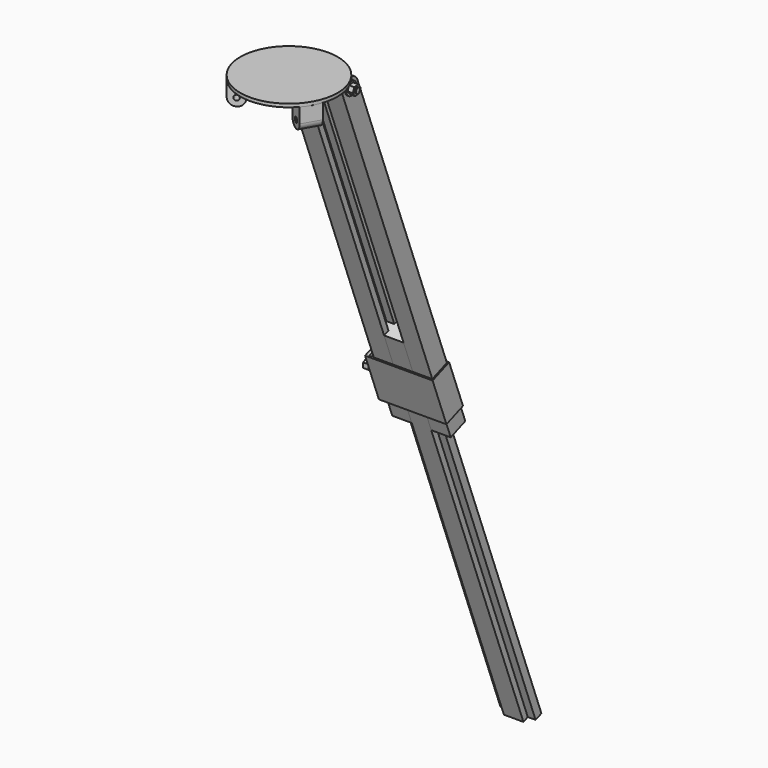
from build123d import *

# Parameters (mm, degrees)
F0_R           = 75
F1_DEPTH       = 5
F2_W           = 30
F2_H           = 24
F3_DEPTH       = 35
F4_R           = 4
F5_DEPTH       = 90.001
F6_R           = 11.99999
F7_COUNT       = 3
F8_R           = 4
F9_DEPTH       = 30
F10_R          = 14.99999
F11_W          = 24
F11_H          = 12
F12_DEPTH      = 570
F15_DEPTH      = 500
F15_DEPTH_BACK = 150
F16_R          = 10
F16_R_2        = 4
F17_DEPTH      = 2
F19_R          = 4
F20_DEPTH      = 104
F22_DEPTH      = 8
F23_R          = 4
F24_DEPTH      = 8
F26_W          = 104
F26_H          = 34
F26_W_2        = 100
F26_H_2        = 30
F27_DEPTH      = 75
F28_W          = 3
F28_H          = 30
F29_DEPTH      = 75
F30_R          = 4
F31_DEPTH      = 9
F32_R          = 7.5
F33_DEPTH      = 2.001
F34_R          = 4
F35_DEPTH      = 7
F35_DEPTH_BACK = 15
F36_R          = 4
F37_DEPTH      = 8
F39_DEPTH      = 8


# Not quite as in the source:
# - a fillet or chamfer is up to 0.001 mm smaller than in the source, because OpenCascade refuses the exact size


with BuildPart() as f1:
    # F0 (on Top) → F1 (new body)
    with BuildSketch(Plane.XY):
        Circle(F0_R)
    extrude(amount=-F1_DEPTH)


with BuildPart() as f3:
    # F2 (on face) → F3 (new body)
    with BuildSketch(Plane(origin=(0, 0, -5), x_dir=(1, 0, 0), z_dir=(0, 0, -1))):
        with Locations((0, -61.4846922835)):
            Rectangle(F2_W, F2_H)
    extrude(amount=F3_DEPTH)

    # F4 (on face) → F5 (cut, through all)
    with BuildSketch(Plane.YZ.offset(15)):
        with Locations((61.4846922835, -28)):
            Circle(F4_R)
    extrude(amount=-F5_DEPTH, mode=Mode.SUBTRACT)

    # F6 (radius 12 in the source; OpenCascade refuses exactly that, so slightly less here)
    f6_edges = [f3.edges().sort_by_distance(p)[0] for p in [
        (0, 49.484692, -40),
        (0, 73.484692, -40),
    ]]
    fillet(f6_edges, radius=F6_R)


with BuildPart() as f7_1:
    # F7: instance of F3
    add(f3.part.rotate(Axis((0, 0, -5), (0, 0, 1)), 1 * 360 / F7_COUNT))


with BuildPart() as f7_2:
    # F7: instance of F3
    add(f3.part.rotate(Axis((0, 0, -5), (0, 0, 1)), 2 * 360 / F7_COUNT))


with BuildPart() as f9:
    # F8 (on face) → F9 (new body)
    with BuildSketch(Plane(origin=(-15, 0, 0), x_dir=(0, -1, 0), z_dir=(-1, 0, 0))):
        Polygon((-42.1390310424, -19.2968171831), (-70.1878751004, -8.6543387589), (-283.0374435832, -569.6312199195), (-254.9885995252, -580.2736983437), align=None)
        with Locations((-61.4846922835, -28)):
            Circle(F8_R, mode=Mode.SUBTRACT)
    extrude(amount=F9_DEPTH)

    # F10 (radius 15 in the source; OpenCascade refuses exactly that, so slightly less here)
    f10_edges = [f9.edges().sort_by_distance(p)[0] for p in [
        (-30, 70.187875, -8.654339),
        (-30, 42.139031, -19.296817),
    ]]
    fillet(f10_edges, radius=F10_R)

    # F11 (on face) → F12 (cut)
    with BuildSketch(Plane(origin=(0, 224.5529499918, -591.8217943299), x_dir=(1, 0, 0), z_dir=(0, 0.3547492808, -0.9349614686))):
        with Locations((-15, -47.5528383313)):
            Rectangle(F11_W, F11_H)
    extrude(amount=-F12_DEPTH, mode=Mode.SUBTRACT)


with BuildPart() as f13_1:
    # F13: instance of F9
    add(f9.part.mirror(Plane.YZ))


with BuildPart() as f15:
    # F14 (on face) → F15 (new body, two sides)
    with BuildSketch(Plane(origin=(0, 224.5529499918, -591.8217943299), x_dir=(1, 0, 0), z_dir=(0, 0.3547492808, -0.9349614686))) as f15_sk:
        Polygon((15, -53.5528383313), (27, -53.5528383313), (27, -41.5528383313), (15, -41.5528383313), (15, -32.5528383313), (-15, -32.5528383313), (-15, -41.5528383313), (-27, -41.5528383313), (-27, -53.5528383313), (-15, -53.5528383313), (-15, -62.5528383313), (15, -62.5528383313), align=None)
    extrude(amount=F15_DEPTH)
    extrude(f15_sk.sketch, amount=-F15_DEPTH_BACK)


with BuildPart() as f17:
    # F16 (on face) → F17 (new body)
    with BuildSketch(Plane(origin=(-45, 0, 0), x_dir=(0, -1, 0), z_dir=(-1, 0, 0))):
        with Locations((-61.4846922835, -28)):
            Circle(F16_R)
        with Locations((-61.4846922835, -28)):
            Circle(F16_R_2, mode=Mode.SUBTRACT)
    extrude(amount=F17_DEPTH)


with BuildPart() as f18_1:
    # F18: instance of F17
    add(f17.part.mirror(Plane.YZ))


with BuildPart() as f20:
    # F19 (on face) → F20 (new body)
    with BuildSketch(Plane(origin=(-47, 0, 0), x_dir=(0, -1, 0), z_dir=(-1, 0, 0))):
        with Locations((-61.4846922835, -28)):
            Circle(F19_R)
    extrude(amount=-F20_DEPTH)

    # F21 (on face) → F22 (join)
    with BuildSketch(Plane(origin=(-47, 0, 0), x_dir=(0, -1, 0), z_dir=(-1, 0, 0))):
        Polygon((-65.2374690332, -34.5), (-57.7319155338, -34.5), (-53.979138784, -28), (-57.7319155338, -21.5), (-65.2374690332, -21.5), (-68.990245783, -28), align=None)
    extrude(amount=F22_DEPTH)


with BuildPart() as f24:
    # F23 (on face) → F24 (new body)
    with BuildSketch(Plane.YZ.offset(47)):
        Polygon((66.0137907142, -33.9850313899), (68.932430725, -27.0702013977), (64.4033322942, -21.0851700078), (56.9555938528, -22.0149686101), (54.036953842, -28.9297986023), (58.5660522728, -34.9148299922), align=None)
        with Locations((61.4846922835, -28)):
            Circle(F23_R, mode=Mode.SUBTRACT)
    extrude(amount=F24_DEPTH)


with BuildPart() as f27:
    # F26 (on offset) → F27 (new body)
    with BuildSketch(Plane(origin=(0, 215.6842179717, -568.4477576148), x_dir=(1, 0, 0), z_dir=(0, 0.3547492808, -0.9349614686))):
        with Locations((-5, -47.5528383313)):
            Rectangle(F26_W, F26_H)
        with Locations((-5, -47.5528383313)):
            Rectangle(F26_W_2, F26_H_2, mode=Mode.SUBTRACT)
    extrude(amount=-F27_DEPTH)


with BuildPart() as f29:
    # F28 (on offset) → F29 (new body)
    with BuildSketch(Plane(origin=(0, 215.6842179717, -568.4477576148), x_dir=(1, 0, 0), z_dir=(0, 0.3547492808, -0.9349614686))):
        with Locations((-46.5, -47.5528383313)):
            Rectangle(F28_W, F28_H)
    extrude(amount=-F29_DEPTH)


with BuildPart() as f29b:
    # F28 (on offset) → F29, piece 2 (new body)
    with BuildSketch(Plane(origin=(0, 215.6842179717, -568.4477576148), x_dir=(1, 0, 0), z_dir=(0, 0.3547492808, -0.9349614686))):
        with Locations((-53.5, -47.5528383313)):
            Rectangle(F28_W, F28_H)
    extrude(amount=-F29_DEPTH)


with BuildPart() as f31_tool:
    # F30 (on face) → F31 (new body, through all)
    with BuildSketch(Plane(origin=(-57, 0, 0), x_dir=(0, -1, 0), z_dir=(-1, 0, 0))):
        with Locations((-246.8411915039, -516.517367344)):
            Circle(F30_R)
    extrude(amount=-F31_DEPTH)


with BuildPart() as f27_1:
    add(f27.part)

    # F31: cut by f31_tool
    add(f31_tool.part, mode=Mode.SUBTRACT)

    # F32 (on face) → F33 (cut, through all)
    with BuildSketch(Plane(origin=(-57, 0, 0), x_dir=(0, -1, 0), z_dir=(-1, 0, 0))):
        with Locations((-246.8411915039, -516.517367344)):
            Circle(F32_R)
    extrude(amount=-F33_DEPTH, mode=Mode.SUBTRACT)


with BuildPart() as f29b_1:
    add(f29b.part)

    # F31: cut by f31_tool
    add(f31_tool.part, mode=Mode.SUBTRACT)


with BuildPart() as f35:
    # F34 (on face) → F35 (new body, two sides)
    with BuildSketch(Plane(origin=(-55, 0, 0), x_dir=(0, -1, 0), z_dir=(-1, 0, 0))) as f35_sk:
        with Locations((-246.8411915039, -516.517367344)):
            Circle(F34_R)
    extrude(amount=-F35_DEPTH)
    extrude(f35_sk.sketch, amount=F35_DEPTH_BACK)

    # F38 (on face) → F39 (join)
    with BuildSketch(Plane(origin=(-70, 0, 0), x_dir=(0, -1, 0), z_dir=(-1, 0, 0))):
        Polygon((-240.3411915039, -520.2701440938), (-240.3411915039, -512.7645905943), (-246.8411915039, -509.0118138446), (-253.3411915039, -512.7645905943), (-253.3411915039, -520.2701440938), (-246.8411915039, -524.0229208435), align=None)
    extrude(amount=F39_DEPTH)


with BuildPart() as f37:
    # F36 (on face) → F37 (new body)
    with BuildSketch(Plane(origin=(-55, 0, 0), x_dir=(0, -1, 0), z_dir=(-1, 0, 0))):
        Polygon((-243.348137725, -523.160552471), (-239.3414975325, -516.8138865982), (-242.8345513113, -510.1707014713), (-250.3342452828, -509.8741822171), (-254.3408854753, -516.2208480898), (-250.8478316965, -522.8640332168), align=None)
        with Locations((-246.8411915039, -516.517367344)):
            Circle(F36_R, mode=Mode.SUBTRACT)
    extrude(amount=F37_DEPTH)


solid = Compound([f1.part, f3.part, f7_1.part, f7_2.part, f9.part, f13_1.part, f15.part, f17.part, f18_1.part, f20.part, f24.part, f29.part, f27_1.part, f29b_1.part, f35.part, f37.part])
